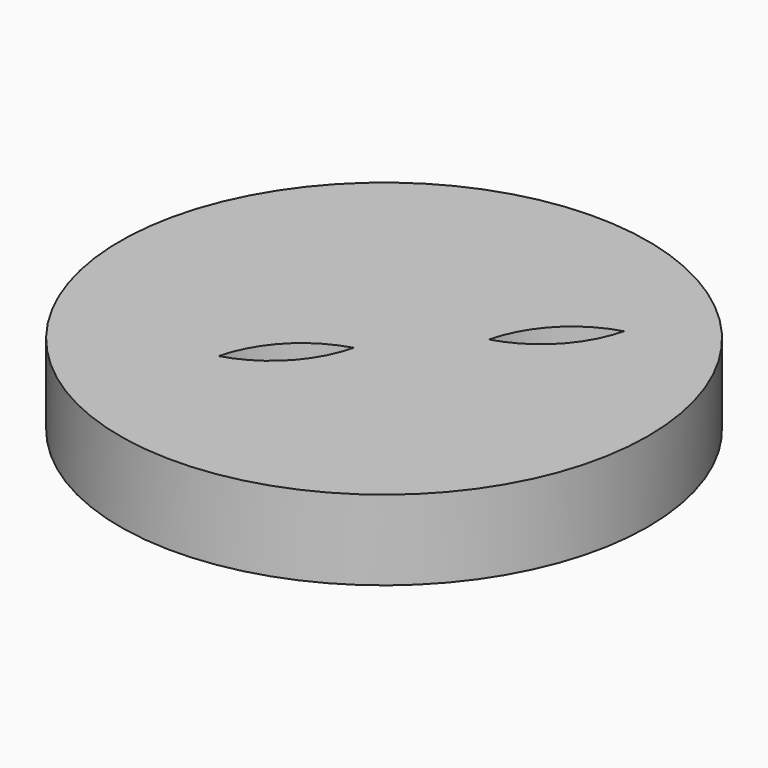
from build123d import *

# Parameters (mm, degrees)
F0_R     = 125.9579420201
F1_DEPTH = 38.1
F3_DEPTH = 38.101


with BuildPart() as f1:
    # F0 (on Top) → F1 (new body)
    with BuildSketch(Plane.XY):
        with Locations((-30.9502501041, -23.8450411707)):
            Circle(F0_R)
    extrude(amount=-F1_DEPTH)

    # F2 (on Top) → F3 (cut, through all)
    with BuildSketch(Plane.XY):
        with BuildLine():
            ThreePointArc((-6.9e-08, -2.01e-08), (22.4870883881, 13.6312603216), (35.1458480619, 36.6798223007))
            ThreePointArc((35.1458480619, 36.6798223007), (12.6587596337, 23.0485619372), (-1.05e-08, -4.28e-08))
        make_face()
        with BuildLine():
            ThreePointArc((-70.2916961239, -73.3596446013), (-47.8046076956, -59.7283842378), (-35.1458480514, -36.6798222578))
            ThreePointArc((-35.1458480539, -36.6798222983), (-57.632936472, -50.3110826452), (-70.2916961239, -73.3596446013))
        make_face()
    extrude(amount=-F3_DEPTH, mode=Mode.SUBTRACT)


solid = f1.part
